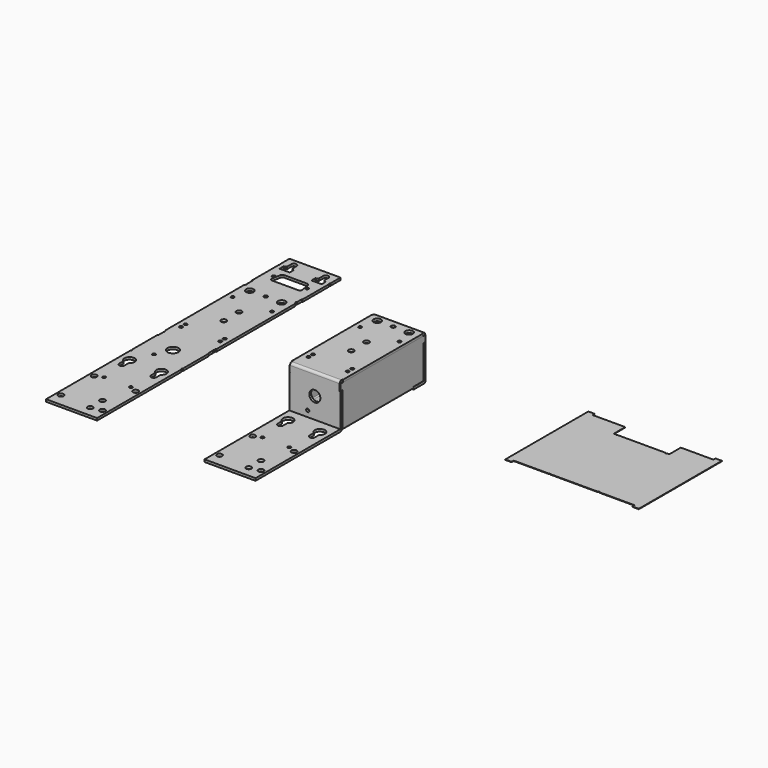
from build123d import *

# Parameters (mm, degrees)
F1_DEPTH       = 25.4
F2_R           = 1.4986
F3_DEPTH       = 2.3622
F4_R           = 2.667
F4_R_2         = 3.81
F4_R_3         = 1.5875
F4_R_4         = 2.0193
F6_DEPTH       = 17.2388907522
F5_R           = 2.667
F5_R_2         = 1.5875
F7_DEPTH       = 2.3622
F8_W           = 10.16
F8_H           = 12.7
F9_DEPTH       = 2.3622
F11_DEPTH      = 48.6338413498
F11_DEPTH_BACK = 57.6905586502
F12_W          = 6.35
F12_H          = 38.1
F12_H_2        = 33.1216
F12_H_3        = 4.9784
F13_DEPTH      = 50.8
F14_W          = 0.635
F14_H          = 12.7
F15_DEPTH      = 3.175
F16_START      = -103.124
F16_DEPTH      = 3.2004
F17_R          = 5.5499
F17_R_2        = 1.5875
F18_DEPTH      = 2.3622
F20_W          = 50.8
F20_H          = 303.149
F21_DEPTH      = 2.286
F23_DEPTH      = 2.286
F24_R          = 2.667
F24_R_2        = 3.81
F24_R_3        = 1.5875
F25_R          = 1.4986
F27_R          = 5.5499
F27_R_2        = 1.5875
F28_R          = 2.667
F28_R_2        = 1.5875
F29_W          = 0.635
F29_H          = 9.779
F30_DEPTH      = 17.2398907522
F32_DEPTH      = 0.2286


with BuildPart() as f1:
    # F0 (on Right) → F1 (new body, symmetric)
    with BuildSketch(Plane.YZ):
        with BuildLine():
            Line((-48.6338413498, -24.8489092478), (-154.2216413498, -24.8489092478))
            Line((-154.2216413498, -24.8489092478), (-154.2216413498, -27.2111092478))
            Line((-154.2216413498, -27.2111092478), (-48.6338413498, -27.2111092478))
            ThreePointArc((-48.6338413498, -27.2111092478), (-46.9635137113, -26.5192368863), (-46.2716413498, -24.8489092478))
            Line((-46.2716413498, -24.8489092478), (-46.2716413498, 14.8766907522))
            Line((-46.2716413498, 14.8766907522), (55.3283586502, 14.8766907522))
            Line((55.3283586502, 14.8766907522), (55.3283586502, -24.8489092478))
            Line((55.3283586502, -24.8489092478), (42.6283586502, -24.8489092478))
            Line((42.6283586502, -24.8489092478), (42.6283586502, -27.2111092478))
            Line((42.6283586502, -27.2111092478), (55.3283586502, -27.2111092478))
            ThreePointArc((55.3283586502, -27.2111092478), (56.9986862887, -26.5192368863), (57.6905586502, -24.8489092478))
            Line((57.6905586502, -24.8489092478), (57.6905586502, 14.8766907522))
            ThreePointArc((57.6905586502, 14.8766907522), (56.9986862887, 16.5470183907), (55.3283586502, 17.2388907522))
            Line((55.3283586502, 17.2388907522), (-46.2716413498, 17.2388907522))
            ThreePointArc((-46.2716413498, 17.2388907522), (-47.9419689883, 16.5470183907), (-48.6338413498, 14.8766907522))
            Line((-48.6338413498, 14.8766907522), (-48.6338413498, -24.8489092478))
        make_face()
    extrude(amount=F1_DEPTH, both=True)

    # F2 (on face) → F3 (cut, through all)
    with BuildSketch(Plane(origin=(0, 57.6905586502, 0), x_dir=(-1, 0, 0), z_dir=(0, 1, 0))):
        with BuildLine():
            Line((-11.5948679627, -14.6635092478), (11.5948679627, -14.6635092478))
            ThreePointArc((11.5948679627, -14.6635092478), (12.9499928015, -14.1702841428), (13.6710396676, -12.921394336))
            Line((13.6710396676, -12.921394336), (15.2206717049, -4.132994336))
            ThreePointArc((15.2206717049, -4.132994336), (14.759474895, -2.4117844091), (13.1445, -1.6587092478))
            Line((13.1445, -1.6587092478), (-13.1445, -1.6587092478))
            ThreePointArc((-13.1445, -1.6587092478), (-14.759474895, -2.4117844091), (-15.2206717049, -4.132994336))
            Line((-15.2206717049, -4.132994336), (-13.6710396676, -12.921394336))
            ThreePointArc((-13.6710396676, -12.921394336), (-12.9499928015, -14.1702841428), (-11.5948679627, -14.6635092478))
        make_face()
        with Locations((16.6878, -8.1611092478)):
            Circle(F2_R)
        with Locations((-16.6878, -8.1611092478)):
            Circle(F2_R)
    extrude(amount=-F3_DEPTH, mode=Mode.SUBTRACT)

    # F4 (on Top) → F6 (cut, through all)
    with BuildSketch(Plane.XY):
        with Locations((0, 15.7805586502)):
            Circle(F4_R)
        with Locations((15.875, 48.9783586502)):
            Circle(F4_R_2)
        with Locations((-15.875, 48.9783586502)):
            Circle(F4_R_2)
        with Locations((19.5453, -32.0984413498)):
            Circle(F4_R_3)
        with Locations((19.5453, 32.2905586502)):
            Circle(F4_R_3)
        with Locations((-19.5453, -32.0984413498)):
            Circle(F4_R_3)
        with Locations((-19.5453, 32.2905586502)):
            Circle(F4_R_3)
        with Locations((0, -3.2694413498)):
            Circle(F4_R)
        with Locations((19.5453, -26.4850413498)):
            Circle(F4_R_3)
        with Locations((-19.5453, -26.4850413498)):
            Circle(F4_R_3)
        with Locations((0, 48.9783586502)):
            Circle(F4_R_4)
    extrude(amount=F6_DEPTH, mode=Mode.SUBTRACT)

    # F5 (on face) → F7 (cut, through all)
    with BuildSketch(Plane.XY.offset(-24.8489092478)):
        with Locations((-20.6375, -141.5216413498)):
            Circle(F5_R)
        with Locations((-20.6375, -100.2466413498)):
            Circle(F5_R)
        with Locations((20.6375, -141.5216413498)):
            Circle(F5_R)
        with Locations((20.6375, -100.2466413498)):
            Circle(F5_R)
        with BuildLine():
            Line((-18.542, 54.1797593394), (-18.542, 48.9783586502))
            ThreePointArc((-18.542, 48.9783586502), (-15.875, 46.3113586502), (-13.208, 48.9783586502))
            Line((-13.208, 48.9783586502), (-13.208, 54.1797593394))
            ThreePointArc((-13.208, 54.1797593394), (-15.875, 63.5833586502), (-18.542, 54.1797593394))
        make_face()
        with BuildLine():
            Line((-13.208, -71.6716413498), (-13.208, -66.4702406606))
            ThreePointArc((-13.208, -66.4702406606), (-15.875, -57.0666413498), (-18.542, -66.4702406606))
            Line((-18.542, -66.4702406606), (-18.542, -71.6716413498))
            ThreePointArc((-18.542, -71.6716413498), (-15.875, -74.3386413498), (-13.208, -71.6716413498))
        make_face()
        with BuildLine():
            Line((18.542, 48.9783586502), (18.542, 54.1797593394))
            ThreePointArc((18.542, 54.1797593394), (15.875, 63.5833586502), (13.208, 54.1797593394))
            Line((13.208, 54.1797593394), (13.208, 48.9783586502))
            ThreePointArc((13.208, 48.9783586502), (15.875, 46.3113586502), (18.542, 48.9783586502))
        make_face()
        with BuildLine():
            Line((18.542, -71.6716413498), (18.542, -66.4702406606))
            ThreePointArc((18.542, -66.4702406606), (15.875, -57.0666413498), (13.208, -66.4702406606))
            Line((13.208, -66.4702406606), (13.208, -71.6716413498))
            ThreePointArc((13.208, -71.6716413498), (15.875, -74.3386413498), (18.542, -71.6716413498))
        make_face()
        with Locations((10.3124, -143.7441413498)):
            Circle(F5_R)
        with Locations((10.3124, -128.5041413498)):
            Circle(F5_R)
        with Locations((-13.335, -97.0716413498)):
            Circle(F5_R_2)
        with Locations((13.335, -97.0716413498)):
            Circle(F5_R_2)
    extrude(amount=-F7_DEPTH, mode=Mode.SUBTRACT)

    # F8 (on face) → F9 (cut, through all)
    with BuildSketch(Plane(origin=(0, 57.6905586502, 0), x_dir=(-1, 0, 0), z_dir=(0, 1, 0))):
        with Locations((-15.875, -27.2111092478)):
            Rectangle(F8_W, F8_H)
        with Locations((15.875, -27.2111092478)):
            Rectangle(F8_W, F8_H)
    extrude(amount=-F9_DEPTH, mode=Mode.SUBTRACT)

    # F14 (on face) → F15 (cut)
    with BuildSketch(Plane(origin=(0, 57.6905586502, 0), x_dir=(-1, 0, 0), z_dir=(0, 1, 0))):
        with Locations((-25.0825, 14.6226907522)):
            Rectangle(F14_W, F14_H)
        with Locations((25.0825, 14.6226907522)):
            Rectangle(F14_W, F14_H)
    extrude(amount=-F15_DEPTH, mode=Mode.SUBTRACT)

    # F14 (on face) → F16 (cut)
    with BuildSketch(Plane(origin=(0, 57.6905586502, 0), x_dir=(-1, 0, 0), z_dir=(0, 1, 0)).offset(F16_START)):
        with Locations((-25.0825, 14.6226907522)):
            Rectangle(F14_W, F14_H)
        with Locations((25.0825, 14.6226907522)):
            Rectangle(F14_W, F14_H)
    extrude(amount=-F16_DEPTH, mode=Mode.SUBTRACT)

    # F17 (on face) → F18 (cut, through all)
    with BuildSketch(Plane.XZ.offset(48.6338413498)):
        with Locations((0, -4.1733092478)):
            Circle(F17_R)
        with Locations((-7.112, -18.9053092478)):
            Circle(F17_R_2)
    extrude(amount=-F18_DEPTH, mode=Mode.SUBTRACT)


with BuildPart() as f11:
    # F10 (on Front) → F11 (new body, two sides)
    with BuildSketch(Plane.XZ) as f11_sk:
        with BuildLine():
            Line((25.4, -25.1791092478), (25.4, 14.8766907522))
            Line((25.4, 14.8766907522), (24.892, 14.8766907522))
            Line((24.892, 14.8766907522), (24.892, -25.1791092478))
            ThreePointArc((24.892, -25.1791092478), (24.5944204897, -25.8975297375), (23.876, -26.1951092478))
            Line((23.876, -26.1951092478), (-23.876, -26.1951092478))
            ThreePointArc((-23.876, -26.1951092478), (-24.5944204897, -25.8975297375), (-24.892, -25.1791092478))
            Line((-24.892, -25.1791092478), (-24.892, 14.8766907522))
            Line((-24.892, 14.8766907522), (-25.4, 14.8766907522))
            Line((-25.4, 14.8766907522), (-25.4, -25.1791092478))
            ThreePointArc((-25.4, -25.1791092478), (-24.9536307345, -26.2567399823), (-23.876, -26.7031092478))
            Line((-23.876, -26.7031092478), (23.876, -26.7031092478))
            ThreePointArc((23.876, -26.7031092478), (24.9536307345, -26.2567399823), (25.4, -25.1791092478))
        make_face()
    extrude(amount=F11_DEPTH)
    extrude(f11_sk.sketch, amount=-F11_DEPTH_BACK)

    # F12 (on face) → F13 (cut, through all)
    with BuildSketch(Plane(origin=(-25.4, 0, 0), x_dir=(0, -1, 0), z_dir=(-1, 0, 0))):
        with Locations((49.1926413498, -10.5233092478)):
            Rectangle(F12_W, F12_H)
        with Locations((-58.2493586502, -8.0341092478)):
            Rectangle(F12_W, F12_H_2)
        with Locations((-58.2493586502, -27.0841092478)):
            Rectangle(F12_W, F12_H_3)
        Polygon((-42.3743586502, -24.5949092478), (-55.0743586502, -24.5949092478), (-55.0743586502, -29.5733092478), (-61.4243586502, -29.5733092478), (-61.4243586502, -30.9449092478), (-42.3743586502, -30.9449092478), align=None)
    extrude(amount=-F13_DEPTH, mode=Mode.SUBTRACT)


with BuildPart() as f21:
    # F20 (on Top) → F21 (new body)
    with BuildSketch(Plane.XY):
        with Locations((-127, -41.2623)):
            Rectangle(F20_W, F20_H)
    extrude(amount=F21_DEPTH)

    # F22 (on Top) → F23 (cut, through all)
    with BuildSketch(Plane.XY):
        Polygon((-99.187, 93.8022), (-99.187, 100.1522), (-102.362, 96.9772), align=None)
        Polygon((-99.822, 52.8066), (-99.822, 59.1566), (-102.997, 55.9816), align=None)
        Polygon((-99.822, -50.0634), (-99.822, -43.7134), (-102.997, -46.8884), align=None)
        Polygon((-99.187, -89.789), (-99.187, -83.439), (-102.362, -86.614), align=None)
        Polygon((-154.178, -50.0634), (-151.003, -46.8884), (-154.178, -43.7134), align=None)
        Polygon((-154.813, 100.1522), (-154.813, 93.8022), (-151.638, 96.9772), align=None)
        Polygon((-154.178, 59.1566), (-154.178, 52.8066), (-151.003, 55.9816), align=None)
        Polygon((-154.813, -83.439), (-154.813, -89.789), (-151.638, -86.614), align=None)
    extrude(amount=F23_DEPTH, mode=Mode.SUBTRACT)

    # F24 (on Top) + F25 (on Top) + F26 (on Top) + F27 (on Top) + F28 (on Top) + F29 (on Top) → F30 (cut, through all)
    with BuildSketch(Plane.XY):
        with Locations((-127, 15.7988)):
            Circle(F24_R)
        with BuildLine():
            ThreePointArc((-114.9339259937, 48.9966), (-111.1239259937, 45.1866), (-107.3139259937, 48.9966))
            ThreePointArc((-107.3139259937, 48.9966), (-111.1239259937, 52.8066), (-114.9339259937, 48.9966))
        make_face()
        with Locations((-142.8760740063, 48.9966)):
            Circle(F24_R_2)
        with BuildLine():
            ThreePointArc((-128.905, 48.9966), (-127, 47.0916), (-125.095, 48.9966))
            Line((-125.095, 48.9966), (-128.905, 48.9966))
        make_face()
        with BuildLine():
            Line((-128.905, 48.9966), (-125.095, 48.9966))
            ThreePointArc((-125.095, 48.9966), (-127, 50.9016), (-128.905, 48.9966))
        make_face()
        with Locations((-107.4547, -32.0802)):
            Circle(F24_R_3)
        with Locations((-107.4547, 32.3088)):
            Circle(F24_R_3)
        with Locations((-146.5453, -32.0802)):
            Circle(F24_R_3)
        with Locations((-146.5453, 32.3088)):
            Circle(F24_R_3)
        with Locations((-127, -3.2512)):
            Circle(F24_R)
        with Locations((-107.4547, -26.4668)):
            Circle(F24_R_3)
        with Locations((-146.5453, -26.4668)):
            Circle(F24_R_3)
    with BuildSketch(Plane.XY):
        with BuildLine():
            Line((-115.4051320373, 86.1568), (-138.5948679627, 86.1568))
            ThreePointArc((-138.5948679627, 86.1568), (-139.9499928015, 85.663574895), (-140.6710396676, 84.4146850882))
            Line((-140.6710396676, 84.4146850882), (-142.2206717049, 75.6262850882))
            ThreePointArc((-142.2206717049, 75.6262850882), (-141.759474895, 73.9050751613), (-140.1445, 73.152))
            Line((-140.1445, 73.152), (-113.8555, 73.152))
            ThreePointArc((-113.8555, 73.152), (-112.240525105, 73.9050751613), (-111.7793282951, 75.6262850882))
            Line((-111.7793282951, 75.6262850882), (-113.3289603324, 84.4146850882))
            ThreePointArc((-113.3289603324, 84.4146850882), (-114.0500071985, 85.663574895), (-115.4051320373, 86.1568))
        make_face()
        with Locations((-143.6878, 79.6544)):
            Circle(F25_R)
        with Locations((-110.3122, 79.6544)):
            Circle(F25_R)
    with BuildSketch(Plane.XY):
        with BuildLine():
            Line((-108.458, 98.7607993108), (-108.458, 103.9622))
            ThreePointArc((-108.458, 103.9622), (-111.125, 106.6292), (-113.792, 103.9622))
            Line((-113.792, 103.9622), (-113.792, 98.7607993108))
            ThreePointArc((-113.792, 98.7607993108), (-114.4906468415, 98.2423046422), (-115.090573729, 97.6122))
            Line((-115.090573729, 97.6122), (-116.205, 97.6122))
            Line((-116.205, 97.6122), (-116.205, 92.3544))
            Line((-116.205, 92.3544), (-106.045, 92.3544))
            Line((-106.045, 92.3544), (-106.045, 97.6122))
            Line((-106.045, 97.6122), (-107.159426271, 97.6122))
            ThreePointArc((-107.159426271, 97.6122), (-107.7593531585, 98.2423046422), (-108.458, 98.7607993108))
        make_face()
        with BuildLine():
            Line((-145.542, 103.9622), (-145.542, 98.7607993108))
            ThreePointArc((-145.542, 98.7607993108), (-146.2406468415, 98.2423046422), (-146.840573729, 97.6122))
            Line((-146.840573729, 97.6122), (-147.955, 97.6122))
            Line((-147.955, 97.6122), (-147.955, 92.3544))
            Line((-147.955, 92.3544), (-137.795, 92.3544))
            Line((-137.795, 92.3544), (-137.795, 97.6122))
            Line((-137.795, 97.6122), (-138.909426271, 97.6122))
            ThreePointArc((-138.909426271, 97.6122), (-139.5093531585, 98.2423046422), (-140.208, 98.7607993108))
            Line((-140.208, 98.7607993108), (-140.208, 103.9622))
            ThreePointArc((-140.208, 103.9622), (-142.875, 106.6292), (-145.542, 103.9622))
        make_face()
    with BuildSketch(Plane.XY):
        with Locations((-127, -66.5734)):
            Circle(F27_R)
        with Locations((-134.112, -81.3054)):
            Circle(F27_R_2)
    with BuildSketch(Plane.XY):
        with Locations((-147.6375, -180.1368)):
            Circle(F28_R)
        with Locations((-106.3625, -180.1368)):
            Circle(F28_R)
        with BuildLine():
            Line((-140.208, -110.2868), (-140.208, -105.0853993108))
            ThreePointArc((-140.208, -105.0853993108), (-142.875, -95.6818), (-145.542, -105.0853993108))
            Line((-145.542, -105.0853993108), (-145.542, -110.2868))
            ThreePointArc((-145.542, -110.2868), (-142.875, -112.9538), (-140.208, -110.2868))
        make_face()
        with BuildLine():
            Line((-108.458, -110.2868), (-108.458, -105.0853993108))
            ThreePointArc((-108.458, -105.0853993108), (-111.125, -95.6818), (-113.792, -105.0853993108))
            Line((-113.792, -105.0853993108), (-113.792, -110.2868))
            ThreePointArc((-113.792, -110.2868), (-111.125, -112.9538), (-108.458, -110.2868))
        make_face()
        with Locations((-116.6876, -182.3593)):
            Circle(F28_R)
        with Locations((-116.6876, -167.1193)):
            Circle(F28_R)
        with Locations((-140.335, -135.6868)):
            Circle(F28_R_2)
        with Locations((-113.665, -135.6868)):
            Circle(F28_R_2)
        with Locations((-147.6375, -138.8618)):
            Circle(F28_R)
        with Locations((-106.3625, -138.8618)):
            Circle(F28_R)
    with BuildSketch(Plane.XY):
        with Locations((-152.0825, -49.2379)):
            Rectangle(F29_W, F29_H)
        with Locations((-101.9175, -49.2379)):
            Rectangle(F29_W, F29_H)
        with Locations((-152.0825, 58.3311)):
            Rectangle(F29_W, F29_H)
        with Locations((-101.9175, 58.3311)):
            Rectangle(F29_W, F29_H)
    extrude(amount=F30_DEPTH, mode=Mode.SUBTRACT)


with BuildPart() as f32:
    # F31 (on Top) → F32 (new body, symmetric)
    with BuildSketch(Plane.XY):
        Polygon((193.802, 57.6905586502), (187.452, 57.6905586502), (187.452, -45.8144413498), (193.802, -45.8144413498), (193.802, -43.1982413498), (228.6, -43.1982413498), (229.362, -42.4362413498), (230.124, -43.1982413498), (277.876, -43.1982413498), (278.638, -42.4362413498), (279.4, -43.1982413498), (314.198, -43.1982413498), (314.198, -45.8144413498), (320.548, -45.8144413498), (320.548, 57.6905586502), (314.198, 57.6905586502), (314.198, 55.0743586502), (281.686, 55.0743586502), (281.686, 40.8503586502), (279.4, 40.8503586502), (278.638, 40.0883586502), (277.876, 40.8503586502), (230.124, 40.8503586502), (229.362, 40.0883586502), (228.6, 40.8503586502), (226.314, 40.8503586502), (226.314, 55.0743586502), (193.802, 55.0743586502), align=None)
    extrude(amount=F32_DEPTH, both=True)


solid = Compound([f1.part, f11.part, f21.part, f32.part])
